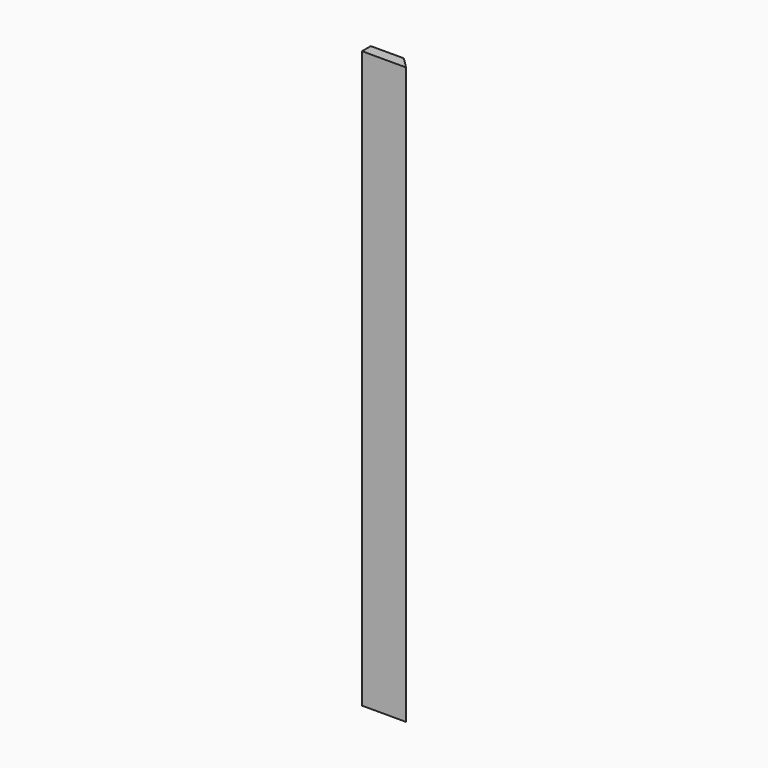
from build123d import *

# Parameters (mm, degrees)
F0_W     = 76.2
F0_H     = 19.05
F1_DEPTH = 498.475
F2_SIZE2 = 19.04999
F2_SIZE  = 19.04999


# Not quite as in the source:
# - a fillet or chamfer is up to 0.001 mm smaller than in the source, because OpenCascade refuses the exact size


with BuildPart() as f1:
    # F0 (on Top) → F1 (new body, symmetric)
    with BuildSketch(Plane.XY):
        Rectangle(F0_W, F0_H)
    extrude(amount=F1_DEPTH, both=True)

    # F2 (size 19.05 and 19.05 in the source; OpenCascade refuses exactly that, so slightly less here)
    f2_edges = [f1.edges().sort_by_distance(p)[0] for p in [
        (38.1, 9.525, 0),
    ]]
    chamfer(f2_edges, length=F2_SIZE, length2=F2_SIZE2)


solid = f1.part
